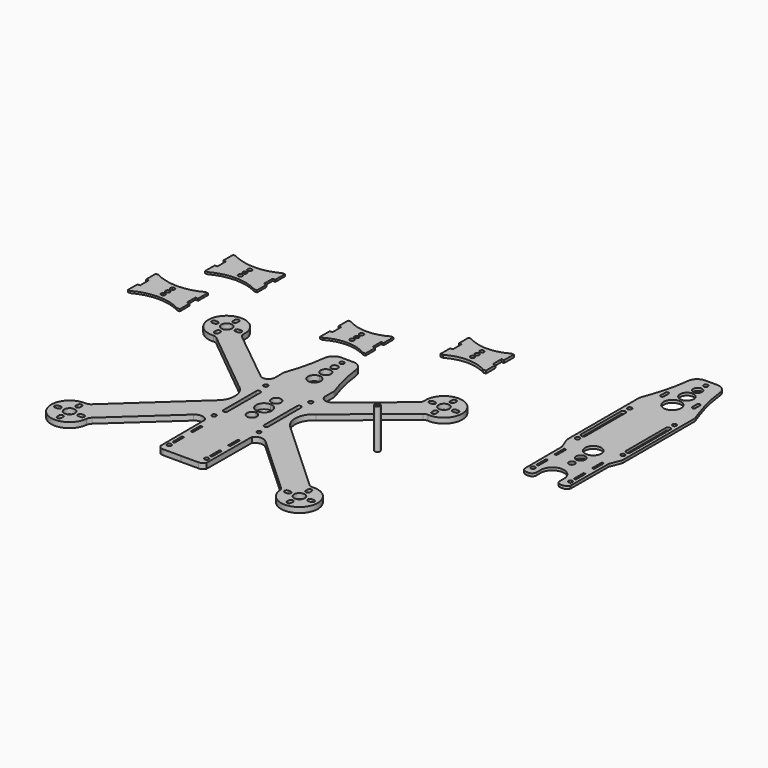
from build123d import *

# Parameters (mm, degrees)
F0_W      = 2
F0_H      = 9.1
F3_DEPTH  = 1.5
F4_W      = 2
F4_H      = 9.1
F5_DEPTH  = 2
F2_R      = 1.5875
F2_W      = 1.6002
F2_H      = 9.125
F6_DEPTH  = 2
F1_R      = 4
F1_R_2    = 1.5875
F7_DEPTH  = 4
F8_R      = 2
F8_R_2    = 1.3
F9_DEPTH  = 30
F10_W     = 2
F10_H     = 9.1
F11_DEPTH = 1.5
F12_W     = 2
F12_H     = 9.1
F13_DEPTH = 1.5


# Not quite as in the source:
# - ends of sketch curves that miss each other by under 0.0002 mm in the source are joined


with BuildPart() as f3:
    # F0 (on Top) → F3 (new body)
    with BuildSketch(Plane.XY):
        with BuildLine():
            Line((-44.4664459562, 44.7763409459), (-57.9039463685, 44.7763409459))
            Line((-57.9039463685, 44.7763409459), (-57.9039463685, 40.7740757426))
            Line((-57.9039463685, 40.7740757426), (-57.9039463685, 31.6763409459))
            ThreePointArc((-57.9039463685, 31.6763409459), (-42.9039463685, 35.7117386538), (-27.9039463685, 31.6763409459))
            Line((-27.9039463685, 31.6763409459), (-27.9039463685, 40.7740757426))
            Line((-27.9039463685, 40.7740757426), (-27.9039463685, 44.7763409459))
            Line((-27.9039463685, 44.7763409459), (-41.3414467807, 44.7763409459))
            ThreePointArc((-41.3414467807, 44.7763409459), (-41.7994933789, 43.6722203901), (-42.9039463685, 43.2149759459))
            ThreePointArc((-42.9039463685, 43.2149759459), (-44.0083993581, 43.6722203901), (-44.4664459562, 44.7763409459))
        make_face()
        with BuildLine():
            ThreePointArc((-42.9039463685, 38.8387946912), (-44.4664463685, 40.4012946912), (-42.9039463685, 41.9637946912))
            ThreePointArc((-42.9039463685, 41.9637946912), (-41.3414463685, 40.4012946912), (-42.9039463685, 38.8387946912))
        make_face(mode=Mode.SUBTRACT)
        with BuildLine():
            ThreePointArc((-27.9039463685, 57.8763409459), (-42.9039463685, 53.840943238), (-57.9039463685, 57.8763409459))
            Line((-57.9039463685, 57.8763409459), (-57.9039463685, 48.7763409459))
            Line((-57.9039463685, 48.7763409459), (-57.9039463685, 44.7763409459))
            Line((-57.9039463685, 44.7763409459), (-44.4664459562, 44.7763409459))
            ThreePointArc((-44.4664459562, 44.7763409459), (-44.0092019243, 45.8819289355), (-42.9039463685, 46.3399759459))
            ThreePointArc((-42.9039463685, 46.3399759459), (-41.7986908126, 45.8819289355), (-41.3414467807, 44.7763409459))
            Line((-41.3414467807, 44.7763409459), (-27.9039463685, 44.7763409459))
            Line((-27.9039463685, 44.7763409459), (-27.9039463685, 48.7763409459))
            Line((-27.9039463685, 48.7763409459), (-27.9039463685, 57.8763409459))
        make_face()
        with BuildLine():
            ThreePointArc((-42.9039463685, 50.8341467508), (-41.3414463685, 49.2716467508), (-42.9039463685, 47.7091467508))
            ThreePointArc((-42.9039463685, 47.7091467508), (-44.4664463685, 49.2716467508), (-42.9039463685, 50.8341467508))
        make_face(mode=Mode.SUBTRACT)
        with Locations((-26.9039463685, 53.3263409459)):
            Rectangle(F0_W, F0_H)
        Polygon((-25.9039463685, 40.7740757426), (-27.9039463685, 40.7740757426), (-27.9039463685, 31.6763409459), (-27.9039463685, 31.6740757426), (-25.9039463685, 31.6740757426), align=None)
        with Locations((-58.9039463685, 53.3263409459)):
            Rectangle(F0_W, F0_H)
        Polygon((-57.9039463685, 31.6763409459), (-57.9039463685, 40.7740757426), (-59.9039463685, 40.7740757426), (-59.9039463685, 31.6740757426), align=None)
    extrude(amount=F3_DEPTH)


with BuildPart() as f5:
    # F4 (on Top) → F5 (new body)
    with BuildSketch(Plane.XY):
        with BuildLine():
            ThreePointArc((41.3305214981, 84.1898763973), (26.3305214981, 80.1544786894), (11.3305214981, 84.1898763973))
            Line((11.3305214981, 84.1898763973), (11.3305214981, 75.0898763973))
            Line((11.3305214981, 75.0898763973), (11.3305214981, 71.0898763973))
            Line((11.3305214981, 71.0898763973), (24.7680219104, 71.0898763973))
            ThreePointArc((24.7680219104, 71.0898763973), (25.2252659423, 72.1954643869), (26.3305214981, 72.6535113973))
            ThreePointArc((26.3305214981, 72.6535113973), (27.435777054, 72.1954643869), (27.8930210859, 71.0898763973))
            Line((27.8930210859, 71.0898763973), (41.3305214981, 71.0898763973))
            Line((41.3305214981, 71.0898763973), (41.3305214981, 75.0898763973))
            Line((41.3305214981, 75.0898763973), (41.3305214981, 84.1898763973))
        make_face()
        with BuildLine():
            ThreePointArc((26.3305214981, 77.1476822022), (27.8930214981, 75.5851822022), (26.3305214981, 74.0226822022))
            ThreePointArc((26.3305214981, 74.0226822022), (24.7680214981, 75.5851822022), (26.3305214981, 77.1476822022))
        make_face(mode=Mode.SUBTRACT)
        with BuildLine():
            Line((24.7680219104, 71.0898763973), (11.3305214981, 71.0898763973))
            Line((11.3305214981, 71.0898763973), (11.3305214981, 67.087611194))
            Line((11.3305214981, 67.087611194), (11.3305214981, 57.9898763973))
            ThreePointArc((11.3305214981, 57.9898763973), (26.3305214981, 62.0252741052), (41.3305214981, 57.9898763973))
            Line((41.3305214981, 57.9898763973), (41.3305214981, 67.087611194))
            Line((41.3305214981, 67.087611194), (41.3305214981, 71.0898763973))
            Line((41.3305214981, 71.0898763973), (27.8930210859, 71.0898763973))
            ThreePointArc((27.8930210859, 71.0898763973), (27.4349744877, 69.9857558415), (26.3305214981, 69.5285113973))
            ThreePointArc((26.3305214981, 69.5285113973), (25.2260685085, 69.9857558415), (24.7680219104, 71.0898763973))
        make_face()
        with BuildLine():
            ThreePointArc((26.3305214981, 65.1523301426), (24.7680214981, 66.7148301426), (26.3305214981, 68.2773301426))
            ThreePointArc((26.3305214981, 68.2773301426), (27.8930214981, 66.7148301426), (26.3305214981, 65.1523301426))
        make_face(mode=Mode.SUBTRACT)
        Polygon((43.3305214981, 67.087611194), (41.3305214981, 67.087611194), (41.3305214981, 57.9898763973), (41.3305214981, 57.987611194), (43.3305214981, 57.987611194), align=None)
        with Locations((42.3305214981, 79.6398763973)):
            Rectangle(F4_W, F4_H)
        with Locations((10.3305214981, 79.6398763973)):
            Rectangle(F4_W, F4_H)
        Polygon((11.3305214981, 57.9898763973), (11.3305214981, 67.087611194), (9.3305214981, 67.087611194), (9.3305214981, 57.987611194), align=None)
    extrude(amount=F5_DEPTH)


with BuildPart() as f6:
    # F2 (on Top) → F6 (new body)
    with BuildSketch(Plane.XY):
        with BuildLine():
            Line((155.8763528676, 128.4774524202), (155.876246806, 128.4774524202))
            Line((155.876246806, 128.4774524202), (155.8761407443, 128.4774523998))
            Line((155.8761407443, 128.4774524202), (151.3094100886, 128.4774524202))
            ThreePointArc((151.3094100886, 128.4774524202), (146.4127010934, 126.6167403622), (143.9873656319, 121.9737072753))
            ThreePointArc((143.9873656319, 121.9737072753), (141.4366050173, 107.6108511655), (137.2573015197, 93.6347487897))
            Line((137.2573015197, 93.6347487897), (135.1935563122, 87.8591692184))
            ThreePointArc((135.1935563122, 87.8591692184), (135.0530988776, 87.3255692993), (135.0058168173, 86.7758224745))
            Line((135.0058168173, 86.7758224745), (135.0058168173, 19.9100591445))
            ThreePointArc((135.0058168173, 19.9100591445), (135.060963688, 19.3167136901), (135.2245151263, 18.743694552))
            Line((135.2245151263, 18.743694552), (138.1936514036, 11.1045397683))
            ThreePointArc((138.1936514036, 11.1045397683), (138.3556602367, 10.5396894348), (138.4123067823, 9.9548014711))
            Line((138.4123067823, 9.9548014711), (138.5925678775, -24.9512348722))
            ThreePointArc((138.5925678775, -24.9512348722), (140.1852851433, -26.826426264), (142.5436343491, -27.5273400025))
            Line((142.5436343491, -27.5273400025), (143.8996695078, -27.5273400025))
            ThreePointArc((143.8996695078, -27.5273400025), (146.1762594456, -26.5843455743), (147.1192538738, -24.3077556365))
            Line((147.1192538738, -24.3077556365), (147.1192538738, -20.6247556365))
            ThreePointArc((147.1192538738, -20.6247556365), (149.5794377566, -14.2301788079), (155.8897137171, -11.5611837055))
            ThreePointArc((155.8897137171, -11.5611837055), (162.2005028923, -14.2289650945), (164.6619166073, -20.6230686343))
            Line((164.6619166073, -20.6230686343), (164.6626249637, -24.3060685662))
            ThreePointArc((164.6626249637, -24.3060685662), (165.6060572341, -26.5824770945), (167.8828284972, -27.5250336456))
            Line((167.8828284972, -27.5250336456), (169.2388636308, -27.5247728375))
            ThreePointArc((169.2388636308, -27.5247728375), (171.5970779853, -26.8234055275), (173.1894345635, -24.9479078408))
            Line((173.1894345635, -24.9479078408), (173.3629821298, 9.9581625267))
            ThreePointArc((173.3629821298, 9.9581625267), (173.419516182, 10.5430613745), (173.5814163737, 11.1079428569))
            Line((173.5814163737, 11.1079428569), (176.5490833471, 18.7476685573))
            ThreePointArc((176.5490833471, 18.7476685573), (176.7125245728, 19.3207191409), (176.7675573235, 19.9140751908))
            Line((176.7675573235, 19.9140751908), (176.75469694, 86.7798372841))
            ThreePointArc((176.75469694, 86.7798372841), (176.707309147, 87.3295750049), (176.566749087, 87.8631478997))
            Line((176.566749087, 87.8631478997), (174.5018930926, 93.6383304413))
            ThreePointArc((174.5018930926, 93.6383304413), (170.3199016294, 107.6136287475), (167.7663786343, 121.9759940003))
            ThreePointArc((167.7663786343, 121.9759940003), (165.3401502168, 126.6185605332), (160.4430834388, 128.4783307661))
            Line((160.4430834388, 128.4783307661), (155.8763528676, 128.4774524405))
        make_face()
        with Locations((141.8560239264, -20.8835245555)):
            Circle(F2_R, mode=Mode.SUBTRACT)
        with Locations((141.8121739264, -12.3689241031)):
            Rectangle(F2_W, F2_H, mode=Mode.SUBTRACT)
        with Locations((141.8121739264, 4.7560758969)):
            Rectangle(F2_W, F2_H, mode=Mode.SUBTRACT)
        with Locations((138.9069576182, 24.590704959)):
            Circle(F2_R, mode=Mode.SUBTRACT)
        with BuildLine():
            ThreePointArc((137.3194112546, 67.0549892372), (139.055853514, 68.7740672747), (140.7575203822, 67.0205591086))
            Line((140.7575203822, 67.0205591086), (140.7578639328, 33.6104760546))
            Line((140.7578639328, 33.6104760546), (140.7578639328, 29.88865924))
            ThreePointArc((140.7578639328, 29.88865924), (139.0386515777, 28.1694424664), (137.3194303855, 29.8886504028))
            Line((137.3194303855, 29.8886504028), (137.3194112546, 33.6104406975))
            Line((137.3194112546, 33.6104406975), (137.3194112546, 67.0549892372))
        make_face(mode=Mode.SUBTRACT)
        with BuildLine():
            ThreePointArc((155.8890146168, -4.2914356483), (153.6566095072, -2.0721551798), (155.8885877383, 0.1475546091))
            ThreePointArc((155.8885877383, 0.1475546091), (158.1209928479, -2.0717258593), (155.8890146168, -4.2914356483))
        make_face(mode=Mode.SUBTRACT)
        with BuildLine():
            ThreePointArc((155.8883440274, 2.6818353952), (152.4370678505, 6.1205559329), (155.8876825898, 9.5599401956))
            ThreePointArc((155.8876825898, 9.5599401956), (159.3389587667, 6.1212196579), (155.8883440274, 2.6818353952))
        make_face(mode=Mode.SUBTRACT)
        with Locations((169.9251962268, -20.8808252644)):
            Circle(F2_R, mode=Mode.SUBTRACT)
        Polygon((170.7833763753, -7.7891995153), (170.7939351549, -16.9141934064), (169.1937362262, -16.9160450403), (169.1831774466, -7.7910511492), align=None, mode=Mode.SUBTRACT)
        Polygon((169.1633616547, 9.3339373861), (170.7635605834, 9.33578902), (170.774119363, 0.2107951289), (169.1739204343, 0.208943495), align=None, mode=Mode.SUBTRACT)
        with BuildLine():
            ThreePointArc((155.887452897, 11.9484512722), (149.8388017165, 17.9959392192), (155.8862896635, 24.0445903996))
            ThreePointArc((155.8862896635, 24.0445903996), (161.9349408439, 17.9971024527), (155.887452897, 11.9484512722))
        make_face(mode=Mode.SUBTRACT)
        with Locations((172.8655163598, 24.593970607)):
            Circle(F2_R, mode=Mode.SUBTRACT)
        with BuildLine():
            Line((174.4448954802, 67.0585594347), (174.4513279159, 33.6140115137))
            Line((174.4513279159, 33.6140115137), (174.452024602, 29.8922212841))
            ThreePointArc((174.452024602, 29.8922212841), (172.7331341001, 28.1726783007), (171.0135911167, 29.8915688027))
            Line((171.0135911167, 29.8915688027), (171.0128752946, 33.6133855484))
            Line((171.0128752946, 33.6133855484), (171.0067930382, 67.0234680505))
            ThreePointArc((171.0067930382, 67.0234680505), (172.7081226203, 68.7773034681), (174.4448954802, 67.0585594347))
        make_face(mode=Mode.SUBTRACT)
        with Locations((139.0386355169, 73.1351176697)):
            Circle(F2_R, mode=Mode.SUBTRACT)
        with BuildLine():
            ThreePointArc((145.2786560799, 101.8923559826), (145.2789936045, 101.8634246129), (145.2786560799, 101.8344932432))
            Line((145.2786560799, 101.8344932432), (145.2786560799, 97.5675112372))
            ThreePointArc((145.2786560799, 97.5675112372), (144.0533460411, 96.2985500188), (142.7987651392, 97.5385798675))
            Line((142.7987651392, 97.5385798675), (142.7987651392, 101.8634246129))
            ThreePointArc((142.7987651392, 101.8634246129), (144.0244127026, 103.1034544616), (145.2786560799, 101.8923559826))
        make_face(mode=Mode.SUBTRACT)
        with BuildLine():
            ThreePointArc((155.8803682862, 85.6193339205), (149.3345290592, 92.1782157718), (155.8791066864, 98.738356472))
            ThreePointArc((155.8791066864, 98.738356472), (162.4249459134, 92.1794746207), (155.8803682862, 85.6193339205))
        make_face(mode=Mode.SUBTRACT)
        with BuildLine():
            ThreePointArc((155.8789190085, 100.6899668871), (150.7560297607, 105.8118709374), (155.8779338109, 110.9347601852))
            ThreePointArc((155.8779338109, 110.9347601852), (161.0008230587, 105.8128561349), (155.8789190085, 100.6899668871))
        make_face(mode=Mode.SUBTRACT)
        with BuildLine():
            ThreePointArc((155.8777775383, 112.5597952039), (152.5637159996, 115.8732194059), (155.8771402016, 119.1872809446))
            ThreePointArc((155.8771402016, 119.1872809446), (159.1912017404, 115.8738567426), (155.8777775383, 112.5597952039))
        make_face(mode=Mode.SUBTRACT)
        with BuildLine():
            ThreePointArc((155.8776198499, 121.8899531092), (155.8768802972, 121.8899525924), (155.8761407443, 121.8899524202))
            ThreePointArc((155.8761407443, 121.8899524202), (154.2886407443, 123.4774524202), (155.8761407443, 125.0649524202))
            ThreePointArc((155.8761407443, 125.0649524202), (155.8765749713, 125.0649523608), (155.8770091982, 125.0649521826))
            ThreePointArc((155.8770091982, 125.0649521826), (157.464814495, 123.4777578591), (155.8776198499, 121.8899531092))
        make_face(mode=Mode.SUBTRACT)
        with Locations((172.7245018504, 73.1383570941)):
            Circle(F2_R, mode=Mode.SUBTRACT)
        with BuildLine():
            Line((166.4797822871, 97.569550058), (166.4789616126, 101.836531985))
            ThreePointArc((166.4789616126, 101.836531985), (166.4786185237, 101.8654632893), (166.4789504838, 101.8943947234))
            ThreePointArc((166.4789504838, 101.8943947234), (167.7329609058, 103.1057344103), (168.9588469431, 101.865940315))
            Line((168.9588469431, 101.865940315), (168.9596787464, 97.5410956496))
            ThreePointArc((168.9596787464, 97.5410956496), (167.7053363643, 96.3008245286), (166.4797822871, 97.569550058))
        make_face(mode=Mode.SUBTRACT)
    extrude(amount=F6_DEPTH)


with BuildPart() as f7:
    # F1 (on Top) → F7 (new body)
    with BuildSketch(Plane.XY):
        with BuildLine():
            Line((55.4423254621, -122.5938338167), (0.8312747552, -72.31776433))
            ThreePointArc((0.8312747552, -72.31776433), (-3.5713049649, -60.9524483755), (2.7441297755, -50.5280347721))
            Line((2.7441297755, -50.5280347721), (51.3242171863, -10.8932593465))
            ThreePointArc((51.3242171863, -10.8932593465), (52.7416112401, -10.1252404704), (54.3419180454, -9.9306202585))
            ThreePointArc((54.3419180454, -9.9306202585), (64.9351919977, 13.5546172758), (41.5501281912, 2.7420030758))
            ThreePointArc((41.5501281912, 2.7420030758), (41.2088558578, 0.7019316724), (39.9579419517, -0.945360814))
            Line((39.9579419517, -0.945360814), (0.7025146083, -32.6546178727))
            ThreePointArc((0.7025146083, -32.6546178727), (0.5270704544, -32.8033856058), (0.3447342931, -32.9436211712))
            ThreePointArc((0.3447342931, -32.9436211712), (-4.4980122119, -33.4435704761), (-7.3103707873, -29.4695571065))
            Line((-7.3103707873, -29.4695571065), (-7.3103707873, -21.2279371224))
            ThreePointArc((-7.3103707873, -21.2279371224), (-7.359671037, -20.6666688157), (-7.506061955, -20.1225894777))
            ThreePointArc((-7.506061955, -20.1225894777), (-11.7540587598, -6.0107609715), (-14.3386475919, 8.4981701128))
            ThreePointArc((-14.3386475919, 8.4981701128), (-16.7639830534, 13.1412031997), (-21.6606920486, 15.0019152577))
            Line((-21.6606920486, 15.0019152577), (-21.8785842975, 15.0019152577))
            Line((-21.8785842975, 15.0019152577), (-26.2273166427, 15.0019152577))
            Line((-26.2273166427, 15.0019152577), (-26.2274227043, 15.0019152577))
            Line((-26.2274227, 15.0019152577), (-26.2275287659, 15.0019152577))
            Line((-26.2275287659, 15.0019152578), (-30.5762611111, 15.0019211709))
            Line((-30.5762611111, 15.0019211709), (-30.7941533515, 15.0019214672))
            ThreePointArc((-30.7941533515, 15.0019214672), (-35.6908648767, 13.1412160673), (-38.1162066515, 8.4981862783))
            ThreePointArc((-38.1162066515, 8.4981862783), (-40.7008152117, -6.0107412918), (-44.9488312046, -20.1225640219))
            ThreePointArc((-44.9488312046, -20.1225640219), (-45.0952228624, -20.6666431607), (-45.1445238753, -21.2279114005))
            Line((-45.1445238753, -21.2279114005), (-45.1445350817, -29.4695313845))
            ThreePointArc((-45.1445350817, -29.4695313845), (-47.9568990637, -33.4435409315), (-52.7996448913, -32.9435850363))
            ThreePointArc((-52.7996448913, -32.9435850363), (-52.9819808591, -32.8033492249), (-53.157424808, -32.6545812554))
            Line((-53.1574248114, -32.6545812596), (-92.4128090441, -0.9452708203))
            ThreePointArc((-92.4128090441, -0.9452708203), (-93.6637207103, 0.7020233671), (-94.0049902698, 2.7420952345))
            ThreePointArc((-94.0049902698, 2.7420952345), (-117.3900393741, 13.5547412317), (-106.7967973552, -9.9305107065))
            ThreePointArc((-106.7967973552, -9.9305107065), (-105.1964908146, -10.1251330944), (-103.7790978051, -10.8931538978))
            Line((-103.7790978051, -10.8931538978), (-55.1990642866, -50.5279953787))
            ThreePointArc((-55.1990642866, -50.5279953787), (-48.8836437205, -60.9524175694), (-53.2862388943, -72.3177275376))
            Line((-53.2862388943, -72.3177275376), (-107.8973579627, -122.5937227683))
            ThreePointArc((-107.8973579627, -122.5937227683), (-109.6107464229, -123.6269577519), (-111.5920541618, -123.9056945287))
            ThreePointArc((-111.5920541618, -123.9056945287), (-122.9110206968, -146.5408303371), (-98.756834306, -138.9881052472))
            ThreePointArc((-98.756834306, -138.9881052472), (-98.2529376891, -137.2450612479), (-97.1601953583, -135.7966040057))
            Line((-97.1601953583, -135.7966040057), (-53.1895755998, -95.4842191234))
            ThreePointArc((-53.1895755998, -95.4842191234), (-48.3264853126, -93.815903761), (-43.7964935435, -96.2473843514))
            ThreePointArc((-43.7964935435, -96.2473843514), (-43.7450638141, -96.3412440629), (-43.7269025606, -96.446718379))
            Line((-43.7269025606, -96.446718379), (-43.51109813, -138.4267485338))
            ThreePointArc((-43.51109813, -138.4267485338), (-41.9183834139, -140.3019420913), (-39.5600351612, -141.0028590364))
            Line((-39.5600351612, -141.0028590364), (-26.2275287659, -141.0028771649))
            Line((-26.2275287659, -141.0028771649), (-12.8950223707, -141.0028771649))
            ThreePointArc((-12.8950223707, -141.0028771649), (-10.5366731649, -140.3019634265), (-8.9439558991, -138.4267720346))
            Line((-8.9439558991, -138.4267720346), (-8.7280943872, -96.4467421734))
            ThreePointArc((-8.7280943872, -96.4467421734), (-8.7099329903, -96.3412678819), (-8.6585031333, -96.2474082404))
            ThreePointArc((-8.6585031333, -96.2474082404), (-4.1285080581, -93.8159338094), (0.7345799607, -95.4842557844))
            Line((0.7345799607, -95.4842557844), (44.7051449055, -135.7967004544))
            ThreePointArc((44.7051449055, -135.7967004544), (45.7978852668, -137.2451591825), (46.3017795137, -138.988203867))
            ThreePointArc((46.3017795137, -138.988203867), (70.4559556348, -146.5409617999), (59.1370198774, -123.9058106008))
            ThreePointArc((59.1370198774, -123.9058106008), (57.1557125175, -123.62707113), (55.4423254621, -122.5938338167))
        make_face()
        with BuildLine():
            Line((-114.039597116, -147.1295236826), (-114.0395949405, -145.5295236826))
            ThreePointArc((-114.0395949405, -145.5295236826), (-112.4395927649, -143.9295258581), (-110.8395949405, -145.5295280337))
            Line((-110.8395949405, -145.5295280337), (-110.839597116, -147.1295280337))
            ThreePointArc((-110.839597116, -147.1295280337), (-112.4395992916, -148.7295258581), (-114.039597116, -147.1295236826))
        make_face(mode=Mode.SUBTRACT)
        with BuildLine():
            ThreePointArc((-122.0395863742, -139.2295128048), (-123.6395841987, -137.6295106292), (-122.0395820231, -136.0295128048))
            Line((-122.0395820231, -136.0295128048), (-120.4395820231, -136.0295149804))
            ThreePointArc((-120.4395820231, -136.0295149804), (-118.8395841987, -137.6295171559), (-120.4395863742, -139.2295149803))
            Line((-120.4395863742, -139.2295149803), (-122.0395863742, -139.2295128048))
        make_face(mode=Mode.SUBTRACT)
        with Locations((-112.4395841987, -137.6295258581)):
            Circle(F1_R, mode=Mode.SUBTRACT)
        with BuildLine():
            ThreePointArc((-104.4395863742, -139.2295367359), (-106.0395841987, -137.6295345604), (-104.4395820231, -136.0295367359))
            Line((-104.4395820231, -136.0295367359), (-102.8395820231, -136.0295389115))
            ThreePointArc((-102.8395820231, -136.0295389115), (-101.2395841987, -137.629541087), (-102.8395863742, -139.2295389115))
            Line((-102.8395863742, -139.2295389115), (-104.4395863742, -139.2295367359))
        make_face(mode=Mode.SUBTRACT)
        with BuildLine():
            ThreePointArc((-114.0395712813, -128.1295236826), (-112.4395691057, -126.5295258581), (-110.8395712813, -128.1295280337))
            Line((-110.8395712813, -128.1295280337), (-110.8395734569, -129.7295280337))
            ThreePointArc((-110.8395734569, -129.7295280337), (-112.4395756324, -131.3295258581), (-114.0395734569, -129.7295236826))
            Line((-114.0395734569, -129.7295236826), (-114.0395712813, -128.1295236826))
        make_face(mode=Mode.SUBTRACT)
        with Locations((-40.2476365481, -134.3575674396)):
            Circle(F1_R_2, mode=Mode.SUBTRACT)
        Polygon((-39.4913811763, -130.4069432304), (-41.0915811763, -130.4069410545), (-41.0915687689, -121.2819410546), (-39.4913687689, -121.2819432304), align=None, mode=Mode.SUBTRACT)
        Polygon((-39.4913578911, -113.2819432304), (-41.0915578911, -113.2819410546), (-41.0915454836, -104.1569410546), (-39.4913454836, -104.1569432304), align=None, mode=Mode.SUBTRACT)
        with Locations((-43.064958687, -88.83576076)):
            Circle(F1_R_2, mode=Mode.SUBTRACT)
        with Locations((-12.207411948, -134.357586503)):
            Circle(F1_R_2, mode=Mode.SUBTRACT)
        Polygon((-11.363488763, -121.2819410546), (-11.3634763555, -130.4069410545), (-12.9636763555, -130.4069432304), (-12.963688763, -121.2819432304), align=None, mode=Mode.SUBTRACT)
        with BuildLine():
            Line((58.3845312536, -147.1296430826), (58.3845312536, -145.5296430826))
            ThreePointArc((58.3845312536, -145.5296430826), (59.9845312536, -143.9296430826), (61.5845312536, -145.5296430826))
            Line((61.5845312536, -145.5296430826), (61.5845312536, -147.1296430826))
            ThreePointArc((61.5845312536, -147.1296430826), (59.9845312536, -148.7296430826), (58.3845312536, -147.1296430826))
        make_face(mode=Mode.SUBTRACT)
        with BuildLine():
            Line((50.3845312536, -136.0296430826), (51.9845312536, -136.0296430826))
            ThreePointArc((51.9845312536, -136.0296430826), (53.5845312536, -137.6296430826), (51.9845312536, -139.2296430826))
            Line((51.9845312536, -139.2296430826), (50.3845312536, -139.2296430826))
            ThreePointArc((50.3845312536, -139.2296430826), (48.7845312536, -137.6296430826), (50.3845312536, -136.0296430826))
        make_face(mode=Mode.SUBTRACT)
        with Locations((59.9845312536, -137.6296430826)):
            Circle(F1_R, mode=Mode.SUBTRACT)
        with BuildLine():
            Line((67.9845312536, -136.0296430826), (69.5845312536, -136.0296430826))
            ThreePointArc((69.5845312536, -136.0296430826), (71.1845312536, -137.6296430826), (69.5845312536, -139.2296430826))
            Line((69.5845312536, -139.2296430826), (67.9845312536, -139.2296430826))
            ThreePointArc((67.9845312536, -139.2296430826), (66.3845312536, -137.6296430826), (67.9845312536, -136.0296430826))
        make_face(mode=Mode.SUBTRACT)
        with BuildLine():
            Line((61.5845312536, -128.1296430826), (61.5845312536, -129.7296430826))
            ThreePointArc((61.5845312536, -129.7296430826), (59.9845312536, -131.3296430826), (58.3845312536, -129.7296430826))
            Line((58.3845312536, -129.7296430826), (58.3845312536, -128.1296430826))
            ThreePointArc((58.3845312536, -128.1296430826), (59.9845312536, -126.5296430826), (61.5845312536, -128.1296430826))
        make_face(mode=Mode.SUBTRACT)
        Polygon((-11.3635120482, -104.1569410546), (-11.3634996407, -113.2819410546), (-12.9636996407, -113.2819432304), (-12.9637120482, -104.1569432304), align=None, mode=Mode.SUBTRACT)
        with Locations((-9.390027912, -88.8357836543)):
            Circle(F1_R_2, mode=Mode.SUBTRACT)
        with BuildLine():
            ThreePointArc((-26.2274859928, -78.0884044908), (-29.9104989964, -74.4054019869), (-26.2274809849, -70.7224044909))
            ThreePointArc((-26.2274809849, -70.7224044909), (-22.5444679813, -74.4054069948), (-26.2274859928, -78.0884044908))
        make_face(mode=Mode.SUBTRACT)
        with BuildLine():
            Line((-43.0649509726, -79.9457608638), (-43.0608459045, -49.4593622105))
            ThreePointArc((-43.0608459045, -49.4593622105), (-43.0649093649, -49.3456362447), (-43.0608152777, -49.2319113774))
            ThreePointArc((-43.0608152777, -49.2319113774), (-41.4782727262, -47.7583502402), (-39.8941283465, -49.2301892044))
            ThreePointArc((-39.8941283465, -49.2301892044), (-39.8899093793, -49.3458521643), (-39.894128661, -49.4615151127))
            Line((-39.8941286549, -49.4615151127), (-39.894169948, -79.830313823))
            ThreePointArc((-39.8941699542, -79.830313823), (-41.4196889346, -81.5324234246), (-43.0649509726, -79.9457608638))
        make_face(mode=Mode.SUBTRACT)
        with Locations((-43.0648927468, -40.3403965985)):
            Circle(F1_R_2, mode=Mode.SUBTRACT)
        with BuildLine():
            Line((-106.1135999626, -4.112378486), (-106.1136021381, -5.712378486))
            ThreePointArc((-106.1136021381, -5.712378486), (-107.7136043137, -7.3123763104), (-109.3136021381, -5.7123741349))
            Line((-109.3136021381, -5.7123741349), (-109.3135999626, -4.1123741349))
            ThreePointArc((-109.3135999626, -4.1123741349), (-107.713597787, -2.5123763104), (-106.1135999626, -4.112378486))
        make_face(mode=Mode.SUBTRACT)
        with BuildLine():
            ThreePointArc((-115.7135870452, 5.3876345673), (-114.1135892208, 3.7876323918), (-115.7135913963, 2.1876345674))
            Line((-115.7135913963, 2.1876345674), (-117.3135913963, 2.1876367429))
            ThreePointArc((-117.3135913963, 2.1876367429), (-118.9135892208, 3.7876389185), (-117.3135870452, 5.3876367429))
            Line((-117.3135870452, 5.3876367429), (-115.7135870452, 5.3876345673))
        make_face(mode=Mode.SUBTRACT)
        with Locations((-107.7135892208, 3.7876236896)):
            Circle(F1_R, mode=Mode.SUBTRACT)
        with BuildLine():
            Line((-109.313578479, 11.6876258651), (-109.3135763034, 13.2876258651))
            ThreePointArc((-109.3135763034, 13.2876258651), (-107.7135741278, 14.8876236896), (-106.1135763034, 13.287621514))
            Line((-106.1135763034, 13.287621514), (-106.113578479, 11.687621514))
            ThreePointArc((-106.113578479, 11.687621514), (-107.7135806545, 10.0876236896), (-109.313578479, 11.6876258651))
        make_face(mode=Mode.SUBTRACT)
        with BuildLine():
            Line((-98.1135913963, 2.1876106362), (-99.7135913963, 2.1876128118))
            ThreePointArc((-99.7135913963, 2.1876128118), (-101.3135892208, 3.7876149873), (-99.7135870452, 5.3876128118))
            Line((-99.7135870452, 5.3876128118), (-98.1135870452, 5.3876106362))
            ThreePointArc((-98.1135870452, 5.3876106362), (-96.5135892208, 3.7876084607), (-98.1135913963, 2.1876106362))
        make_face(mode=Mode.SUBTRACT)
        with BuildLine():
            ThreePointArc((-26.2274717449, -57.1313950416), (-20.358389823, -63.0004849438), (-26.2274797253, -68.8695668657))
            ThreePointArc((-26.2274797253, -68.8695668657), (-32.0965616472, -63.0004769635), (-26.2274717449, -57.1313950416))
        make_face(mode=Mode.SUBTRACT)
        with BuildLine():
            ThreePointArc((-9.3941174711, -49.2319342661), (-9.3900235385, -49.345659139), (-9.3940871535, -49.4593850992))
            Line((-9.3940871535, -49.4593850992), (-9.3900235385, -79.9457837581))
            ThreePointArc((-9.3900235385, -79.9457837581), (-11.0352877339, -81.5324440818), (-12.5608044, -79.8303324059))
            Line((-12.5608044, -79.8303324059), (-12.5608044, -49.4615336956))
            ThreePointArc((-12.5608044, -49.4615336956), (-12.5650235244, -49.3458707412), (-12.5608044, -49.2302077868))
            ThreePointArc((-12.5608044, -49.2302077868), (-10.9766580187, -47.7583709771), (-9.3941174711, -49.2319342661))
        make_face(mode=Mode.SUBTRACT)
        with BuildLine():
            ThreePointArc((-26.2274654774, -47.9125574164), (-22.5444679813, -51.5955599203), (-26.2274704853, -55.2785574164))
            ThreePointArc((-26.2274704853, -55.2785574164), (-29.9104679813, -51.5955549125), (-26.2274654774, -47.9125574164))
        make_face(mode=Mode.SUBTRACT)
        with Locations((-9.390027912, -40.3404194927)):
            Circle(F1_R_2, mode=Mode.SUBTRACT)
        with BuildLine():
            ThreePointArc((-26.2274404616, -11.1171243326), (-21.4699158383, -15.8746554248), (-26.2274469305, -20.6321800481))
            ThreePointArc((-26.2274469305, -20.6321800481), (-30.9849715539, -15.8746489559), (-26.2274404616, -11.1171243326))
        make_face(mode=Mode.SUBTRACT)
        with BuildLine():
            ThreePointArc((-26.2274337429, -1.2346663439), (-22.3490281693, -5.1130771911), (-26.2274390165, -8.9914827647))
            ThreePointArc((-26.2274390165, -8.9914827647), (-30.1058445901, -5.1130719176), (-26.2274337429, -1.2346663439))
        make_face(mode=Mode.SUBTRACT)
        with BuildLine():
            ThreePointArc((-26.227429149, 5.5224765168), (-23.7401115453, 3.0351555311), (-26.2274325311, 0.5478379274))
            ThreePointArc((-26.2274325311, 0.5478379274), (-28.7147501347, 3.0351589131), (-26.227429149, 5.5224765168))
        make_face(mode=Mode.SUBTRACT)
        with BuildLine():
            ThreePointArc((-26.2273255998, 8.4144152707), (-26.2274271829, 8.4144152609), (-26.2275287659, 8.4144152577))
            ThreePointArc((-26.2275287659, 8.4144152708), (-27.8148234413, 10.0019152575), (-26.2275287659, 11.5894152443))
            ThreePointArc((-26.2275287659, 11.5894152577), (-26.2274250243, 11.5894152543), (-26.2273212827, 11.5894152441))
            ThreePointArc((-26.2273212827, 11.5894152441), (-24.6400287659, 10.0019130991), (-26.2273255998, 8.4144152707))
        make_face(mode=Mode.SUBTRACT)
        with BuildLine():
            Line((53.6587285638, -5.712487109), (53.6587285638, -4.112487109))
            ThreePointArc((53.6587285638, -4.112487109), (55.2587285638, -2.512487109), (56.8587285638, -4.112487109))
            Line((56.8587285638, -4.112487109), (56.8587285638, -5.712487109))
            ThreePointArc((56.8587285638, -5.712487109), (55.2587285638, -7.312487109), (53.6587285638, -5.712487109))
        make_face(mode=Mode.SUBTRACT)
        with BuildLine():
            Line((45.6587285638, 5.387512891), (47.2587285638, 5.387512891))
            ThreePointArc((47.2587285638, 5.387512891), (48.8587285638, 3.787512891), (47.2587285638, 2.187512891))
            Line((47.2587285638, 2.187512891), (45.6587285638, 2.187512891))
            ThreePointArc((45.6587285638, 2.187512891), (44.0587285638, 3.787512891), (45.6587285638, 5.387512891))
        make_face(mode=Mode.SUBTRACT)
        with Locations((55.2587285638, 3.787512891)):
            Circle(F1_R, mode=Mode.SUBTRACT)
        with BuildLine():
            Line((63.2587285638, 5.387512891), (64.8587285638, 5.387512891))
            ThreePointArc((64.8587285638, 5.387512891), (66.4587285638, 3.787512891), (64.8587285638, 2.187512891))
            Line((64.8587285638, 2.187512891), (63.2587285638, 2.187512891))
            ThreePointArc((63.2587285638, 2.187512891), (61.6587285638, 3.787512891), (63.2587285638, 5.387512891))
        make_face(mode=Mode.SUBTRACT)
        with BuildLine():
            Line((56.8587285638, 13.287512891), (56.8587285638, 11.687512891))
            ThreePointArc((56.8587285638, 11.687512891), (55.2587285638, 10.087512891), (53.6587285638, 11.687512891))
            Line((53.6587285638, 11.687512891), (53.6587285638, 13.287512891))
            ThreePointArc((53.6587285638, 13.287512891), (55.2587285638, 14.887512891), (56.8587285638, 13.287512891))
        make_face(mode=Mode.SUBTRACT)
    extrude(amount=F7_DEPTH)


with BuildPart() as f9:
    # F8 (on Top) → F9 (new body)
    with BuildSketch(Plane.XY):
        with Locations((54.602060467, -57.8380823135)):
            Circle(F8_R)
        with Locations((54.602060467, -57.8380823135)):
            Circle(F8_R_2, mode=Mode.SUBTRACT)
    extrude(amount=F9_DEPTH)


with BuildPart() as f11:
    # F10 (on Top) → F11 (new body)
    with BuildSketch(Plane.XY):
        with BuildLine():
            ThreePointArc((-127.6205689662, 80.8045635421), (-136.1038902285, 77.5559695059), (-145.1205339662, 76.451325418))
            Line((-145.1205339662, 76.451325418), (-145.1205339662, 73.762369347))
            ThreePointArc((-145.1205339662, 73.762369347), (-143.5580339662, 72.199869347), (-145.1205339662, 70.637369347))
            Line((-145.1205339662, 70.637369347), (-145.1205339662, 69.2681985421))
            ThreePointArc((-145.1205339662, 69.2681985421), (-144.0152784103, 68.8101515317), (-143.5580343784, 67.7045635421))
            Line((-143.5580343784, 67.7045635421), (-127.6205689662, 67.7045635421))
            Line((-127.6205689662, 67.7045635421), (-127.6205689662, 71.7045635421))
            Line((-127.6205689662, 71.7045635421), (-127.6205689662, 80.8045635421))
        make_face()
        with Locations((-163.6204989662, 76.2545635421)):
            Rectangle(F10_W, F10_H)
        with BuildLine():
            ThreePointArc((-145.1205339662, 76.451325418), (-154.1371777038, 77.5559695059), (-162.6204989662, 80.8045635421))
            Line((-162.6204989662, 80.8045635421), (-162.6204989662, 71.7045635421))
            Line((-162.6204989662, 71.7045635421), (-162.6204989662, 67.7045635421))
            Line((-162.6204989662, 67.7045635421), (-146.6830335539, 67.7045635421))
            ThreePointArc((-146.6830335539, 67.7045635421), (-146.225789522, 68.8101515317), (-145.1205339662, 69.2681985421))
            Line((-145.1205339662, 69.2681985421), (-145.1205339662, 70.637369347))
            ThreePointArc((-145.1205339662, 70.637369347), (-146.6830339662, 72.199869347), (-145.1205339662, 73.762369347))
            Line((-145.1205339662, 73.762369347), (-145.1205339662, 76.451325418))
        make_face()
        with BuildLine():
            ThreePointArc((-143.5580343784, 67.7045635421), (-144.0160809766, 66.6004429862), (-145.1205339662, 66.1431985421))
            Line((-145.1205339662, 66.1431985421), (-145.1205339662, 64.8920172874))
            ThreePointArc((-145.1205339662, 64.8920172874), (-143.5580339662, 63.3295172874), (-145.1205339662, 61.7670172874))
            Line((-145.1205339662, 61.7670172874), (-145.1205339662, 58.9812437579))
            ThreePointArc((-145.1205339662, 58.9812437579), (-136.1010535943, 57.8704791393), (-127.6205689662, 54.6045635421))
            Line((-127.6205689662, 54.6045635421), (-127.6205689662, 63.7022983387))
            Line((-127.6205689662, 63.7022983387), (-127.6205689662, 67.7045635421))
            Line((-127.6205689662, 67.7045635421), (-143.5580343784, 67.7045635421))
        make_face()
        Polygon((-125.6205689662, 63.7022983387), (-127.6205689662, 63.7022983387), (-127.6205689662, 54.6045635421), (-127.6205689662, 54.6022983387), (-125.6205689662, 54.6022983387), align=None)
        with Locations((-126.6205689662, 76.2545635421)):
            Rectangle(F10_W, F10_H)
        Polygon((-162.6204989662, 54.6045635421), (-162.6204989662, 63.7022983387), (-164.6204989662, 63.7022983387), (-164.6204989662, 54.6022983387), align=None)
        with BuildLine():
            Line((-146.6830335539, 67.7045635421), (-162.6204989662, 67.7045635421))
            Line((-162.6204989662, 67.7045635421), (-162.6204989662, 63.7022983387))
            Line((-162.6204989662, 63.7022983387), (-162.6204989662, 54.6045635421))
            ThreePointArc((-162.6204989662, 54.6045635421), (-154.140014338, 57.8704791393), (-145.1205339662, 58.9812437579))
            Line((-145.1205339662, 58.9812437579), (-145.1205339662, 61.7670172874))
            ThreePointArc((-145.1205339662, 61.7670172874), (-146.6830339662, 63.3295172874), (-145.1205339662, 64.8920172874))
            Line((-145.1205339662, 64.8920172874), (-145.1205339662, 66.1431985421))
            ThreePointArc((-145.1205339662, 66.1431985421), (-146.2249869558, 66.6004429862), (-146.6830335539, 67.7045635421))
        make_face()
    extrude(amount=F11_DEPTH)


with BuildPart() as f13:
    # F12 (on Top) → F13 (new body)
    with BuildSketch(Plane.XY):
        with BuildLine():
            ThreePointArc((-147.9669716612, 33.8699137749), (-156.4502929235, 30.6213197387), (-165.4669366612, 29.5166756508))
            Line((-165.4669366612, 29.5166756508), (-165.4669366612, 26.8277195798))
            ThreePointArc((-165.4669366612, 26.8277195798), (-163.9044366612, 25.2652195798), (-165.4669366612, 23.7027195798))
            Line((-165.4669366612, 23.7027195798), (-165.4669366612, 22.3335487749))
            ThreePointArc((-165.4669366612, 22.3335487749), (-164.3616811053, 21.8755017645), (-163.9044370734, 20.7699137749))
            Line((-163.9044370734, 20.7699137749), (-147.9669716612, 20.7699137749))
            Line((-147.9669716612, 20.7699137749), (-147.9669716612, 24.7699137749))
            Line((-147.9669716612, 24.7699137749), (-147.9669716612, 33.8699137749))
        make_face()
        with BuildLine():
            ThreePointArc((-165.4669366612, 29.5166756508), (-174.4835803988, 30.6213197387), (-182.9669016612, 33.8699137749))
            Line((-182.9669016612, 33.8699137749), (-182.9669016612, 24.7699137749))
            Line((-182.9669016612, 24.7699137749), (-182.9669016612, 20.7699137749))
            Line((-182.9669016612, 20.7699137749), (-167.0294362489, 20.7699137749))
            ThreePointArc((-167.0294362489, 20.7699137749), (-166.572192217, 21.8755017645), (-165.4669366612, 22.3335487749))
            Line((-165.4669366612, 22.3335487749), (-165.4669366612, 23.7027195798))
            ThreePointArc((-165.4669366612, 23.7027195798), (-167.0294366612, 25.2652195798), (-165.4669366612, 26.8277195798))
            Line((-165.4669366612, 26.8277195798), (-165.4669366612, 29.5166756508))
        make_face()
        with BuildLine():
            Line((-167.0294362489, 20.7699137749), (-182.9669016612, 20.7699137749))
            Line((-182.9669016612, 20.7699137749), (-182.9669016612, 16.7676485716))
            Line((-182.9669016612, 16.7676485716), (-182.9669016612, 7.6699137749))
            ThreePointArc((-182.9669016612, 7.6699137749), (-174.486417033, 10.9358293721), (-165.4669366612, 12.0465939907))
            Line((-165.4669366612, 12.0465939907), (-165.4669366612, 14.8323675202))
            ThreePointArc((-165.4669366612, 14.8323675202), (-167.0294366612, 16.3948675202), (-165.4669366612, 17.9573675202))
            Line((-165.4669366612, 17.9573675202), (-165.4669366612, 19.2085487749))
            ThreePointArc((-165.4669366612, 19.2085487749), (-166.5713896508, 19.6657932191), (-167.0294362489, 20.7699137749))
        make_face()
        Polygon((-182.9669016612, 7.6699137749), (-182.9669016612, 16.7676485716), (-184.9669016612, 16.7676485716), (-184.9669016612, 7.6676485716), align=None)
        Polygon((-145.9669716612, 16.7676485716), (-147.9669716612, 16.7676485716), (-147.9669716612, 7.6699137749), (-147.9669716612, 7.6676485716), (-145.9669716612, 7.6676485716), align=None)
        with Locations((-146.9669716612, 29.3199137749)):
            Rectangle(F12_W, F12_H)
        with Locations((-183.9669016612, 29.3199137749)):
            Rectangle(F12_W, F12_H)
        with BuildLine():
            ThreePointArc((-163.9044370734, 20.7699137749), (-164.3624836715, 19.6657932191), (-165.4669366612, 19.2085487749))
            Line((-165.4669366612, 19.2085487749), (-165.4669366612, 17.9573675202))
            ThreePointArc((-165.4669366612, 17.9573675202), (-163.9044366612, 16.3948675202), (-165.4669366612, 14.8323675202))
            Line((-165.4669366612, 14.8323675202), (-165.4669366612, 12.0465939907))
            ThreePointArc((-165.4669366612, 12.0465939907), (-156.4474562893, 10.9358293721), (-147.9669716612, 7.6699137749))
            Line((-147.9669716612, 7.6699137749), (-147.9669716612, 16.7676485716))
            Line((-147.9669716612, 16.7676485716), (-147.9669716612, 20.7699137749))
            Line((-147.9669716612, 20.7699137749), (-163.9044370734, 20.7699137749))
        make_face()
    extrude(amount=F13_DEPTH)


solid = Compound([f3.part, f5.part, f6.part, f7.part, f9.part, f11.part, f13.part])
